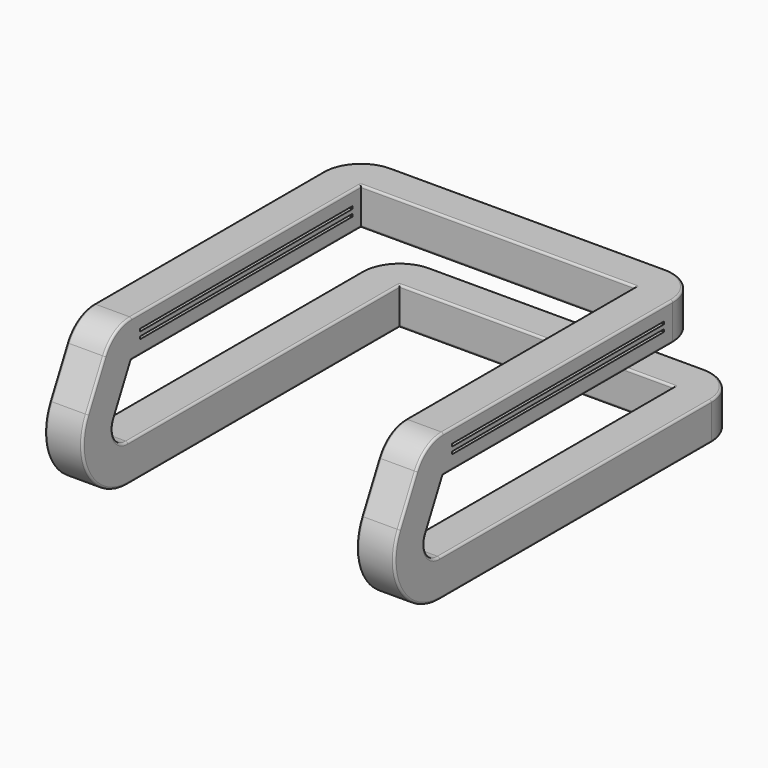
from build123d import *

# Parameters (mm, degrees)
F7_W          = 313.3465600376
F7_H          = 3
F8_DEPTH      = 412.7510001
F8_DEPTH_BACK = 908


# Not quite as in the source:
# - an extrude ends at something that could not be found from the text; its depth is read off the source's solid


with BuildPart() as f5:
    # F5: sweep along a path in F1, F0, F3
    with BuildLine(Plane.XY) as f5_path:
        Line((184.15, 127), (22.225, 127))
        ThreePointArc((22.225, 127), (6.5095517881, 120.4904482119), (0, 104.775))
        Line((0, 104.775), (0, 0))
    with BuildLine(Plane.YZ) as f5_path_2:
        Line((0, 0), (-296.6715600376, 0))
        ThreePointArc((-296.6715600376, 0), (-334.5266189482, 21.1519954744), (-336.3542297256, 64.4771871822))
        Line((-336.3542297256, 64.4771871822), (-310.9628948816, 114.7885935911))
        ThreePointArc((-310.9628948816, 114.7885935911), (-302.7705623004, 123.7025294553), (-291.1215600376, 127))
        Line((-291.1215600376, 127), (-57.15, 127))
    with BuildLine(Plane.XY.offset(127)) as f5_path_3:
        Line((0, -57.15), (0, 47.625))
        ThreePointArc((0, 47.625), (6.5095517881, 63.3404482119), (22.225, 69.85))
        Line((22.225, 69.85), (184.15, 69.85))
    # F4 (on Front) → F5 (sweep)
    with BuildSketch(Plane.XZ):
        with BuildLine():
            Line((-19.725, -22.225), (19.725, -22.225))
            ThreePointArc((19.725, -22.225), (21.492766953, -21.492766953), (22.225, -19.725))
            Line((22.225, -19.725), (22.225, 19.725))
            ThreePointArc((22.225, 19.725), (21.492766953, 21.492766953), (19.725, 22.225))
            Line((19.725, 22.225), (-19.725, 22.225))
            ThreePointArc((-19.725, 22.225), (-21.492766953, 21.492766953), (-22.225, 19.725))
            Line((-22.225, 19.725), (-22.225, -19.725))
            ThreePointArc((-22.225, -19.725), (-21.492766953, -21.492766953), (-19.725, -22.225))
        make_face()
    sweep(path=f5_path.line + f5_path_2.line + f5_path_3.line)

    # F6: F5 across face


with BuildPart() as f5_1:
    add(f5.part)
    add(f5.part.mirror(Plane(origin=(184.15, 127, 0), x_dir=(0, 1, 0), z_dir=(1, 0, 0))))

    # F7 (on face) → F8 (cut, two sides)
    with BuildSketch(Plane(origin=(-22.225, 0, 0), x_dir=(0, -1, 0), z_dir=(-1, 0, 0))) as f8_sk:
        with Locations((121.7482800188, 123)):
            Rectangle(F7_W, F7_H)
        with Locations((121.7482800188, 131)):
            Rectangle(F7_W, F7_H)
    extrude(amount=-F8_DEPTH, mode=Mode.SUBTRACT)
    extrude(f8_sk.sketch, amount=F8_DEPTH_BACK, mode=Mode.SUBTRACT)


solid = f5_1.part
